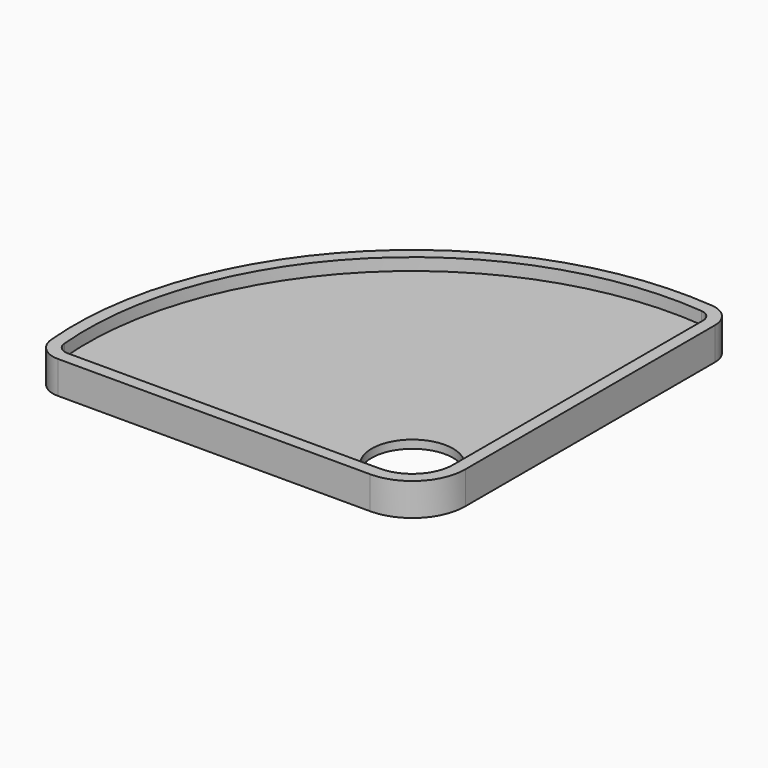
from build123d import *

# Parameters (mm, degrees)
F1_DEPTH = 4
F2_T     = -1.5
F5_DEPTH = 1
F6_R     = 3
F7_R     = 1.5
F9_DEPTH = 25


with BuildPart() as f1:
    # F0 (on Top) → F1 (new body)
    with BuildSketch(Plane.XY):
        with BuildLine():
            ThreePointArc((-6.5, 0), (-1.9038059223, 1.9038059223), (0, 6.5))
            Line((0, 6.5), (0, 47.4878030638))
            ThreePointArc((0, 47.4878030638), (-35.8449314192, 35.8449314192), (-47.4878030638, 0))
            Line((-47.4878030638, 0), (-13, 0))
            Line((-13, 0), (-6.5, 0))
        make_face()
    extrude(amount=F1_DEPTH)

    # F2
    f2_openings = [f1.faces().sort_by_distance(p)[0] for p in [
        (-21.274509, 21.274509, 4),
        (-21.274509, 21.274509, 0),
    ]]
    offset(amount=F2_T, openings=f2_openings)

    # F4 (on offset) → F5 (join)
    with BuildSketch(Plane.XY.offset(1.5)):
        with BuildLine():
            Line((-46.186269666, 1.5), (-6.5, 1.5))
            ThreePointArc((-6.5, 1.5), (-2.9644660941, 2.9644660941), (-1.5, 6.5))
            Line((-1.5, 6.5), (-1.5, 46.186269666))
            ThreePointArc((-1.5, 46.186269666), (-34.7842712475, 34.7842712475), (-46.186269666, 1.5))
        make_face()
    extrude(amount=F5_DEPTH)

    # F6
    f6_edges = [f1.edges().sort_by_distance(p)[0] for p in [
        (0, 47.487803, 2),
        (-47.487803, 0, 2),
    ]]
    fillet(f6_edges, radius=F6_R)

    # F7
    f7_edges = [f1.edges().sort_by_distance(p)[0] for p in [
        (-1.5, 46.18627, 0.75),
        (-46.18627, 1.5, 0.75),
        (-46.18627, 1.5, 3.25),
        (-1.5, 46.18627, 3.25),
    ]]
    fillet(f7_edges, radius=F7_R)

    # F8 (on face) → F9 (cut)
    with BuildSketch(Plane.XY.offset(4)):
        with BuildLine():
            ThreePointArc((-6.5, 1.5), (-2.9644660941, 2.9644660941), (-1.5, 6.5))
            ThreePointArc((-1.5, 6.5), (-10.0355339059, 10.0355339059), (-6.5, 1.5))
        make_face()
    extrude(amount=-F9_DEPTH, mode=Mode.SUBTRACT)


solid = f1.part
